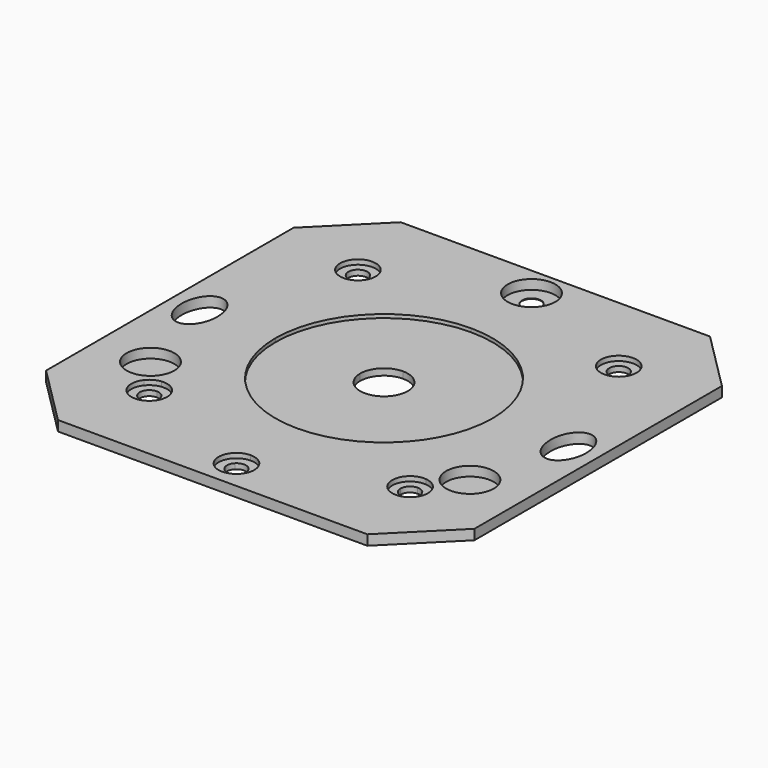
from build123d import *

# Parameters (mm, degrees)
F0_R      = 18.25
F1_DEPTH  = 1.7
F3_DEPTH  = 0.6
F4_R      = 1.6
F4_R_2    = 3
F5_DEPTH  = 0.8
F7_DEPTH  = 25
F8_R      = 2.5
F9_DEPTH  = 1.6
F10_R     = 4
F10_R_2   = 3
F11_DEPTH = 1.6
F13_DEPTH = 0.8
F15_DEPTH = 25


with BuildPart() as f1:
    # F0 (on Top) → F1 (new body)
    with BuildSketch(Plane.XY):
        Polygon((12.8613220751, 42.5075584586), (-39.1386779249, 42.5075584586), (-49.1386779249, 32.5075584586), (-49.1386779249, -19.4924415414), (-39.1386779249, -29.4924415414), (12.8613220751, -29.4924415414), (22.8613220751, -19.4924415414), (22.8613220751, 32.5075584586), align=None)
        with BuildLine():
            ThreePointArc((-35.0589881417, 26.8278686754), (-36.1903589916, 29.5592395253), (-33.4589881417, 28.4278686754))
            Line((-33.4589881417, 28.4278686754), (-22.2183677081, 28.4278686754))
            Line((-22.2183677081, 28.4278686754), (-14.2700487748, 36.3761876087))
            ThreePointArc((-14.2700487748, 36.3761876087), (-13.7509714167, 38.9857657106), (-11.5386779249, 37.5075584586))
            ThreePointArc((-11.5386779249, 37.5075584586), (-11.6604706729, 36.8952649668), (-12.007307075, 36.3761876087))
            Line((-12.007307075, 36.3761876087), (-4.0589881417, 28.4278686754))
            Line((-4.0589881417, 28.4278686754), (7.1816322919, 28.4278686754))
            ThreePointArc((7.1816322919, 28.4278686754), (8.7816322919, 30.0278686754), (10.3816322919, 28.4278686754))
            ThreePointArc((10.3816322919, 28.4278686754), (9.9130031418, 27.2964978255), (8.7816322919, 26.8278686754))
            Line((8.7816322919, 26.8278686754), (8.7816322919, 15.5872482418))
            Line((8.7816322919, 15.5872482418), (16.7299512252, 7.6389293085))
            ThreePointArc((16.7299512252, 7.6389293085), (18.4736155669, 7.9857657106), (19.4613220751, 6.5075584586))
            ThreePointArc((19.4613220751, 6.5075584586), (18.4736155669, 5.0293512066), (16.7299512252, 5.3761876087))
            Line((16.7299512252, 5.3761876087), (8.7816322919, -2.5721313246))
            Line((8.7816322919, -2.5721313246), (8.7816322919, -13.8127517582))
            ThreePointArc((8.7816322919, -13.8127517582), (9.9130031418, -14.2813809083), (10.3816322919, -15.4127517582))
            ThreePointArc((10.3816322919, -15.4127517582), (8.7816322919, -17.0127517582), (7.1816322919, -15.4127517582))
            Line((7.1816322919, -15.4127517582), (-4.0589881417, -15.4127517582))
            Line((-4.0589881417, -15.4127517582), (-12.007307075, -23.3610706915))
            ThreePointArc((-12.007307075, -23.3610706915), (-11.6604706729, -23.8801480496), (-11.5386779249, -24.4924415414))
            ThreePointArc((-11.5386779249, -24.4924415414), (-13.7509714167, -25.9706487934), (-14.2700487748, -23.3610706915))
            Line((-14.2700487748, -23.3610706915), (-22.2183677081, -15.4127517582))
            Line((-22.2183677081, -15.4127517582), (-33.4589881417, -15.4127517582))
            ThreePointArc((-33.4589881417, -15.4127517582), (-36.1903589916, -16.5441226081), (-35.0589881417, -13.8127517582))
            Line((-35.0589881417, -13.8127517582), (-35.0589881417, -2.5721313246))
            Line((-35.0589881417, -2.5721313246), (-43.007307075, 5.3761876087))
            ThreePointArc((-43.007307075, 5.3761876087), (-45.7386779249, 6.5075584586), (-43.007307075, 7.6389293085))
            Line((-43.007307075, 7.6389293085), (-35.0589881417, 15.5872482418))
            Line((-35.0589881417, 15.5872482418), (-35.0589881417, 26.8278686754))
        make_face(mode=Mode.SUBTRACT)
        with BuildLine():
            Line((-22.2183677081, 28.4278686754), (-33.4589881417, 28.4278686754))
            ThreePointArc((-33.4589881417, 28.4278686754), (-33.9276172918, 27.2964978255), (-35.0589881417, 26.8278686754))
            Line((-35.0589881417, 26.8278686754), (-35.0589881417, 15.5872482418))
            Line((-35.0589881417, 15.5872482418), (-22.2183677081, 28.4278686754))
        make_face()
        with BuildLine():
            Line((-14.2700487748, 36.3761876087), (-22.2183677081, 28.4278686754))
            Line((-22.2183677081, 28.4278686754), (-4.0589881417, 28.4278686754))
            Line((-4.0589881417, 28.4278686754), (-12.007307075, 36.3761876087))
            ThreePointArc((-12.007307075, 36.3761876087), (-13.1386779249, 35.9075584586), (-14.2700487748, 36.3761876087))
        make_face()
        with BuildLine():
            Line((7.1816322919, 28.4278686754), (-4.0589881417, 28.4278686754))
            Line((-4.0589881417, 28.4278686754), (8.7816322919, 15.5872482418))
            Line((8.7816322919, 15.5872482418), (8.7816322919, 26.8278686754))
            ThreePointArc((8.7816322919, 26.8278686754), (7.650261442, 27.2964978255), (7.1816322919, 28.4278686754))
        make_face()
        with BuildLine():
            Line((16.7299512252, 7.6389293085), (8.7816322919, 15.5872482418))
            Line((8.7816322919, 15.5872482418), (8.7816322919, -2.5721313246))
            Line((8.7816322919, -2.5721313246), (16.7299512252, 5.3761876087))
            ThreePointArc((16.7299512252, 5.3761876087), (16.2613220751, 6.5075584586), (16.7299512252, 7.6389293085))
        make_face()
        with BuildLine():
            Line((8.7816322919, -13.8127517582), (8.7816322919, -2.5721313246))
            Line((8.7816322919, -2.5721313246), (-4.0589881417, -15.4127517582))
            Line((-4.0589881417, -15.4127517582), (7.1816322919, -15.4127517582))
            ThreePointArc((7.1816322919, -15.4127517582), (7.650261442, -14.2813809083), (8.7816322919, -13.8127517582))
        make_face()
        with BuildLine():
            Line((-4.0589881417, -15.4127517582), (-22.2183677081, -15.4127517582))
            Line((-22.2183677081, -15.4127517582), (-14.2700487748, -23.3610706915))
            ThreePointArc((-14.2700487748, -23.3610706915), (-13.1386779249, -22.8924415414), (-12.007307075, -23.3610706915))
            Line((-12.007307075, -23.3610706915), (-4.0589881417, -15.4127517582))
        make_face()
        with BuildLine():
            Line((-22.2183677081, -15.4127517582), (-35.0589881417, -2.5721313246))
            Line((-35.0589881417, -2.5721313246), (-35.0589881417, -13.8127517582))
            ThreePointArc((-35.0589881417, -13.8127517582), (-33.9276172918, -14.2813809083), (-33.4589881417, -15.4127517582))
            Line((-33.4589881417, -15.4127517582), (-22.2183677081, -15.4127517582))
        make_face()
        with BuildLine():
            Line((-35.0589881417, -2.5721313246), (-35.0589881417, 15.5872482418))
            Line((-35.0589881417, 15.5872482418), (-43.007307075, 7.6389293085))
            ThreePointArc((-43.007307075, 7.6389293085), (-42.6604706729, 7.1198519504), (-42.5386779249, 6.5075584586))
            ThreePointArc((-42.5386779249, 6.5075584586), (-42.6604706729, 5.8952649668), (-43.007307075, 5.3761876087))
            Line((-43.007307075, 5.3761876087), (-35.0589881417, -2.5721313246))
        make_face()
        Polygon((-4.0589881417, 28.4278686754), (-22.2183677081, 28.4278686754), (-35.0589881417, 15.5872482418), (-35.0589881417, -2.5721313246), (-22.2183677081, -15.4127517582), (-4.0589881417, -15.4127517582), (8.7816322919, -2.5721313246), (8.7816322919, 15.5872482418), align=None)
        with Locations((-13.1386779249, 6.5075584586)):
            Circle(F0_R, mode=Mode.SUBTRACT)
        with Locations((-13.1386779249, 6.5075584586)):
            Circle(F0_R)
    extrude(amount=F1_DEPTH)

    # F2 (on face) → F3 (cut)
    with BuildSketch(Plane.XY.offset(1.7)):
        with BuildLine():
            Line((-31.3886779249, 6.5075584586), (-13.1386779249, 6.5075584586))
            Line((-13.1386779249, 6.5075584586), (-13.1386779249, 24.7575584586))
            ThreePointArc((-13.1386779249, 24.7575584586), (-26.0433766815, 19.4122572153), (-31.3886779249, 6.5075584586))
        make_face()
        with BuildLine():
            ThreePointArc((-13.1386779249, -11.7424415414), (-0.2339791682, -6.397140298), (5.1113220751, 6.5075584586))
            Line((5.1113220751, 6.5075584586), (-13.1386779249, 6.5075584586))
            Line((-13.1386779249, 6.5075584586), (-13.1386779249, -11.7424415414))
        make_face()
        with BuildLine():
            Line((-13.1386779249, 6.5075584586), (5.1113220751, 6.5075584586))
            ThreePointArc((5.1113220751, 6.5075584586), (-0.2339791682, 19.4122572153), (-13.1386779249, 24.7575584586))
            Line((-13.1386779249, 24.7575584586), (-13.1386779249, 6.5075584586))
        make_face()
        with BuildLine():
            Line((-13.1386779249, -11.7424415414), (-13.1386779249, 6.5075584586))
            Line((-13.1386779249, 6.5075584586), (-31.3886779249, 6.5075584586))
            ThreePointArc((-31.3886779249, 6.5075584586), (-26.0433766815, -6.397140298), (-13.1386779249, -11.7424415414))
        make_face()
    extrude(amount=-F3_DEPTH, mode=Mode.SUBTRACT)

    # F4 (on face) → F5 (cut)
    with BuildSketch(Plane.XY.offset(1.7)):
        with BuildLine():
            ThreePointArc((-45.7386779249, 6.5075584586), (-44.1386779249, 8.1075584586), (-42.5386779249, 6.5075584586))
            Line((-42.5386779249, 6.5075584586), (-41.1386779249, 6.5075584586))
            ThreePointArc((-41.1386779249, 6.5075584586), (-44.1386779249, 9.5075584586), (-47.1386779249, 6.5075584586))
            Line((-47.1386779249, 6.5075584586), (-45.7386779249, 6.5075584586))
        make_face()
        with BuildLine():
            ThreePointArc((-45.7386779249, 6.5075584586), (-44.1386779249, 4.9075584586), (-42.5386779249, 6.5075584586))
            Line((-42.5386779249, 6.5075584586), (-45.7386779249, 6.5075584586))
        make_face()
        with BuildLine():
            Line((-45.7386779249, 6.5075584586), (-42.5386779249, 6.5075584586))
            ThreePointArc((-42.5386779249, 6.5075584586), (-44.1386779249, 8.1075584586), (-45.7386779249, 6.5075584586))
        make_face()
        with BuildLine():
            Line((-41.1386779249, 6.5075584586), (-42.5386779249, 6.5075584586))
            ThreePointArc((-42.5386779249, 6.5075584586), (-44.1386779249, 4.9075584586), (-45.7386779249, 6.5075584586))
            Line((-45.7386779249, 6.5075584586), (-47.1386779249, 6.5075584586))
            ThreePointArc((-47.1386779249, 6.5075584586), (-44.1386779249, 3.5075584586), (-41.1386779249, 6.5075584586))
        make_face()
        with BuildLine():
            ThreePointArc((-35.4323567059, -9.5934317721), (-36.3209238445, -8.8312520534), (-37.4590547769, -8.5571581567))
            Line((-37.4590547769, -8.5571581567), (-37.4590547769, -11.0571581567))
            Line((-37.4590547769, -11.0571581567), (-35.4323567059, -9.5934317721))
        make_face()
        with BuildLine():
            Line((-37.4590547769, -11.0571581567), (-37.4590547769, -8.5571581567))
            ThreePointArc((-37.4590547769, -8.5571581567), (-39.6849608802, -9.9190272243), (-39.4857528479, -12.5208845413))
            Line((-39.4857528479, -12.5208845413), (-37.4590547769, -11.0571581567))
        make_face()
        with BuildLine():
            Line((-34.9590547769, -11.0571581567), (-37.4590547769, -11.0571581567))
            Line((-37.4590547769, -11.0571581567), (-39.4857528479, -12.5208845413))
            ThreePointArc((-39.4857528479, -12.5208845413), (-38.5779651724, -13.2927877161), (-37.4159766348, -13.5567869839))
            ThreePointArc((-37.4159766348, -13.5567869839), (-36.5068235367, -12.7852486338), (-35.3689396686, -12.4288063748))
            ThreePointArc((-35.3689396686, -12.4288063748), (-35.0637168288, -11.7729487089), (-34.9590547769, -11.0571581567))
        make_face()
        with BuildLine():
            Line((-35.4323567059, -9.5934317721), (-37.4590547769, -11.0571581567))
            Line((-37.4590547769, -11.0571581567), (-34.9590547769, -11.0571581567))
            ThreePointArc((-34.9590547769, -11.0571581567), (-35.0803213768, -10.2879849569), (-35.4323567059, -9.5934317721))
        make_face()
        with BuildLine():
            ThreePointArc((-35.3689396686, -12.4288063748), (-36.5068235367, -12.7852486338), (-37.4159766348, -13.5567869839))
            ThreePointArc((-37.4159766348, -13.5567869839), (-36.252525281, -13.2467440937), (-35.3689396686, -12.4288063748))
        make_face()
        with BuildLine():
            ThreePointArc((-35.3689396686, -12.4288063748), (-36.252525281, -13.2467440937), (-37.4159766348, -13.5567869839))
            ThreePointArc((-37.4159766348, -13.5567869839), (-36.0410865381, -18.2474444646), (-32.0589881417, -15.4127517582))
            ThreePointArc((-32.0589881417, -15.4127517582), (-33.0502391007, -13.1845400783), (-35.3689396686, -12.4288063748))
        make_face()
        with Locations((-35.0589881417, -15.4127517582)):
            Circle(F4_R, mode=Mode.SUBTRACT)
        with BuildLine():
            ThreePointArc((-13.1386779249, 40.5075584586), (-16.1386779249, 37.5075584586), (-13.1386779249, 34.5075584586))
            Line((-13.1386779249, 34.5075584586), (-13.1386779249, 35.9075584586))
            ThreePointArc((-13.1386779249, 35.9075584586), (-14.7386779249, 37.5075584586), (-13.1386779249, 39.1075584586))
            Line((-13.1386779249, 39.1075584586), (-13.1386779249, 40.5075584586))
        make_face()
        with BuildLine():
            Line((-13.1386779249, 35.9075584586), (-13.1386779249, 34.5075584586))
            ThreePointArc((-13.1386779249, 34.5075584586), (-11.0173575813, 35.3862381151), (-10.1386779249, 37.5075584586))
            ThreePointArc((-10.1386779249, 37.5075584586), (-11.0173575813, 39.6288788022), (-13.1386779249, 40.5075584586))
            Line((-13.1386779249, 40.5075584586), (-13.1386779249, 39.1075584586))
            ThreePointArc((-13.1386779249, 39.1075584586), (-12.007307075, 38.6389293085), (-11.5386779249, 37.5075584586))
            ThreePointArc((-11.5386779249, 37.5075584586), (-12.007307075, 36.3761876087), (-13.1386779249, 35.9075584586))
        make_face()
        with BuildLine():
            ThreePointArc((-10.1386779249, -24.4924415414), (-11.0173575813, -22.3711211978), (-13.1386779249, -21.4924415414))
            Line((-13.1386779249, -21.4924415414), (-13.1386779249, -22.8924415414))
            ThreePointArc((-13.1386779249, -22.8924415414), (-12.007307075, -23.3610706915), (-11.5386779249, -24.4924415414))
            ThreePointArc((-11.5386779249, -24.4924415414), (-12.007307075, -25.6238123913), (-13.1386779249, -26.0924415414))
            Line((-13.1386779249, -26.0924415414), (-13.1386779249, -27.4924415414))
            ThreePointArc((-13.1386779249, -27.4924415414), (-11.0173575813, -26.6137618849), (-10.1386779249, -24.4924415414))
        make_face()
        with BuildLine():
            Line((-13.1386779249, -22.8924415414), (-13.1386779249, -21.4924415414))
            ThreePointArc((-13.1386779249, -21.4924415414), (-16.1386779249, -24.4924415414), (-13.1386779249, -27.4924415414))
            Line((-13.1386779249, -27.4924415414), (-13.1386779249, -26.0924415414))
            ThreePointArc((-13.1386779249, -26.0924415414), (-14.7386779249, -24.4924415414), (-13.1386779249, -22.8924415414))
        make_face()
        with BuildLine():
            ThreePointArc((11.1816989271, -8.5571581567), (10.0435679947, -8.8312520534), (9.1550008561, -9.5934317721))
            Line((9.1550008561, -9.5934317721), (11.1816989271, -11.0571581567))
            Line((11.1816989271, -11.0571581567), (11.1816989271, -8.5571581567))
        make_face()
        with BuildLine():
            Line((11.1816989271, -11.0571581567), (9.1550008561, -9.5934317721))
            ThreePointArc((9.1550008561, -9.5934317721), (8.802965527, -10.2879849569), (8.6816989271, -11.0571581567))
            Line((8.6816989271, -11.0571581567), (11.1816989271, -11.0571581567))
        make_face()
        with BuildLine():
            ThreePointArc((20.8613220751, 6.5075584586), (17.8613220751, 9.5075584586), (14.8613220751, 6.5075584586))
            Line((14.8613220751, 6.5075584586), (16.2613220751, 6.5075584586))
            ThreePointArc((16.2613220751, 6.5075584586), (17.8613220751, 8.1075584586), (19.4613220751, 6.5075584586))
            Line((19.4613220751, 6.5075584586), (20.8613220751, 6.5075584586))
        make_face()
        with BuildLine():
            Line((16.2613220751, 6.5075584586), (14.8613220751, 6.5075584586))
            ThreePointArc((14.8613220751, 6.5075584586), (17.8613220751, 3.5075584586), (20.8613220751, 6.5075584586))
            Line((20.8613220751, 6.5075584586), (19.4613220751, 6.5075584586))
            ThreePointArc((19.4613220751, 6.5075584586), (17.8613220751, 4.9075584586), (16.2613220751, 6.5075584586))
        make_face()
        with BuildLine():
            ThreePointArc((13.6816989271, -11.0571581567), (12.9494658801, -9.2893912037), (11.1816989271, -8.5571581567))
            Line((11.1816989271, -8.5571581567), (11.1816989271, -11.0571581567))
            Line((11.1816989271, -11.0571581567), (13.2083969981, -12.5208845413))
            ThreePointArc((13.2083969981, -12.5208845413), (13.5604323272, -11.8263313565), (13.6816989271, -11.0571581567))
        make_face()
        with BuildLine():
            ThreePointArc((11.138620785, -13.5567869839), (10.229467687, -12.7852486338), (9.0915838189, -12.4288063748))
            ThreePointArc((9.0915838189, -12.4288063748), (9.9751694312, -13.2467440937), (11.138620785, -13.5567869839))
        make_face()
        with BuildLine():
            ThreePointArc((11.138620785, -13.5567869839), (9.9751694312, -13.2467440937), (9.0915838189, -12.4288063748))
            ThreePointArc((9.0915838189, -12.4288063748), (6.553420612, -17.4215007991), (11.7816322919, -15.4127517582))
            ThreePointArc((11.7816322919, -15.4127517582), (11.6163249983, -14.4306533617), (11.138620785, -13.5567869839))
        make_face()
        with Locations((8.7816322919, -15.4127517582)):
            Circle(F4_R, mode=Mode.SUBTRACT)
        with BuildLine():
            ThreePointArc((19.4613220751, 6.5075584586), (17.8613220751, 8.1075584586), (16.2613220751, 6.5075584586))
            Line((16.2613220751, 6.5075584586), (19.4613220751, 6.5075584586))
        make_face()
        with BuildLine():
            Line((19.4613220751, 6.5075584586), (16.2613220751, 6.5075584586))
            ThreePointArc((16.2613220751, 6.5075584586), (17.8613220751, 4.9075584586), (19.4613220751, 6.5075584586))
        make_face()
        with Locations((-35.0589881417, 28.4278686754)):
            Circle(F4_R_2)
        with Locations((-35.0589881417, 28.4278686754)):
            Circle(F4_R, mode=Mode.SUBTRACT)
        with Locations((8.7816322919, 28.4278686754)):
            Circle(F4_R_2)
        with Locations((8.7816322919, 28.4278686754)):
            Circle(F4_R, mode=Mode.SUBTRACT)
        with Locations((-35.0589881417, -15.4127517582)):
            Circle(F4_R)
        with Locations((8.7816322919, -15.4127517582)):
            Circle(F4_R)
        with Locations((-35.0589881417, 28.4278686754)):
            Circle(F4_R)
        with Locations((8.7816322919, 28.4278686754)):
            Circle(F4_R)
    extrude(amount=-F5_DEPTH, mode=Mode.SUBTRACT)

    # F6 (on face) → F7 (cut)
    with BuildSketch(Plane.XY.offset(1.7)):
        with BuildLine():
            ThreePointArc((-9.1386779249, 6.5075584586), (-10.3102508001, 9.3359855834), (-13.1386779249, 10.5075584586))
            Line((-13.1386779249, 10.5075584586), (-13.1386779249, 6.5075584586))
            Line((-13.1386779249, 6.5075584586), (-9.1386779249, 6.5075584586))
        make_face()
        with BuildLine():
            Line((-13.1386779249, 6.5075584586), (-13.1386779249, 10.5075584586))
            ThreePointArc((-13.1386779249, 10.5075584586), (-15.9671050496, 9.3359855834), (-17.1386779249, 6.5075584586))
            Line((-17.1386779249, 6.5075584586), (-13.1386779249, 6.5075584586))
        make_face()
        with BuildLine():
            Line((-9.1386779249, 6.5075584586), (-13.1386779249, 6.5075584586))
            Line((-13.1386779249, 6.5075584586), (-13.1386779249, 2.5075584586))
            ThreePointArc((-13.1386779249, 2.5075584586), (-10.3102508001, 3.6791313339), (-9.1386779249, 6.5075584586))
        make_face()
        with BuildLine():
            Line((-13.1386779249, 2.5075584586), (-13.1386779249, 6.5075584586))
            Line((-13.1386779249, 6.5075584586), (-17.1386779249, 6.5075584586))
            ThreePointArc((-17.1386779249, 6.5075584586), (-15.9671050496, 3.6791313339), (-13.1386779249, 2.5075584586))
        make_face()
    extrude(amount=-F7_DEPTH, mode=Mode.SUBTRACT)

    # F8 (on face) → F9 (join)
    with BuildSketch(Plane.XY.offset(1.7)):
        with Locations((-37.4590547769, -11.0571581567)):
            Circle(F8_R)
        with Locations((11.1816989271, -11.0571581567)):
            Circle(F8_R)
    extrude(amount=-F9_DEPTH)

    # F10 (on face) → F11 (cut)
    with BuildSketch(Plane.XY.offset(1.7)):
        with Locations((-13.1386779249, 37.5075584586)):
            Circle(F10_R)
        with Locations((-13.1386779249, 37.5075584586)):
            Circle(F10_R_2, mode=Mode.SUBTRACT)
        with Locations((13.7081095924, -8.9924415414)):
            Circle(F10_R)
        with Locations((-39.9854654422, -8.9924415414)):
            Circle(F10_R)
        with Locations((-44.1386779249, 6.5075584586)):
            Circle(F10_R_2)
        with Locations((-13.1386779249, 37.5075584586)):
            Circle(F10_R_2)
    extrude(amount=-F11_DEPTH, mode=Mode.SUBTRACT)

    # F12 (on face) → F13 (cut)
    with BuildSketch(Plane.XY.offset(1.7)):
        with BuildLine():
            ThreePointArc((9.0915838189, -12.4288063748), (9.9751694312, -13.2467440937), (11.138620785, -13.5567869839))
            ThreePointArc((11.138620785, -13.5567869839), (10.229467687, -12.7852486338), (9.0915838189, -12.4288063748))
        make_face()
        with BuildLine():
            ThreePointArc((9.0915838189, -12.4288063748), (6.553420612, -17.4215007991), (11.7816322919, -15.4127517582))
            ThreePointArc((11.7816322919, -15.4127517582), (11.6163249983, -14.4306533617), (11.138620785, -13.5567869839))
            ThreePointArc((11.138620785, -13.5567869839), (9.9751694312, -13.2467440937), (9.0915838189, -12.4288063748))
        make_face()
        with BuildLine():
            ThreePointArc((-37.4159766348, -13.5567869839), (-36.0410865381, -18.2474444646), (-32.0589881417, -15.4127517582))
            ThreePointArc((-32.0589881417, -15.4127517582), (-33.0502391007, -13.1845400783), (-35.3689396686, -12.4288063748))
            ThreePointArc((-35.3689396686, -12.4288063748), (-36.252525281, -13.2467440937), (-37.4159766348, -13.5567869839))
        make_face()
        with BuildLine():
            ThreePointArc((-37.4159766348, -13.5567869839), (-36.252525281, -13.2467440937), (-35.3689396686, -12.4288063748))
            ThreePointArc((-35.3689396686, -12.4288063748), (-36.5068235367, -12.7852486338), (-37.4159766348, -13.5567869839))
        make_face()
    extrude(amount=-F13_DEPTH, mode=Mode.SUBTRACT)

    # F14 (on face) → F15 (cut)
    with BuildSketch(Plane.XY.offset(1.7)):
        with BuildLine():
            add(Edge.make_bspline(
                [(-47.1386779249, 6.5075585663), (-47.1386779967, 2.0075585125), (-44.1386779608, 2.0075584586), (-41.1386779249, 2.0075584048), (-41.1386779249, 6.5075584586)],
                knots=[1.5707963029, 1.5707963029, 1.5707963029, 3.1415926416, 3.1415926416, 4.7123889804, 4.7123889804, 4.7123889804], degree=2, weights=[1, 0.707106777, 1, 0.707106777, 1]))
            ThreePointArc((-41.1386779249, 6.5075584586), (-44.1386779787, 3.5075584586), (-47.1386779249, 6.5075585663))
        make_face()
        with BuildLine():
            add(Edge.make_bspline(
                [(14.8613220751, 6.5075584586), (14.8613220751, 2.0075584586), (17.8613220751, 2.0075584586), (20.8613220751, 2.0075584586), (20.8613220751, 6.5075584586)],
                knots=[1.5707963268, 1.5707963268, 1.5707963268, 3.1415926536, 3.1415926536, 4.7123889804, 4.7123889804, 4.7123889804], degree=2, weights=[1, 0.7071067812, 1, 0.7071067812, 1]))
            ThreePointArc((20.8613220751, 6.5075584586), (17.8613220751, 3.5075584586), (14.8613220751, 6.5075584586))
        make_face()
        with BuildLine():
            ThreePointArc((14.8613220751, 6.5075584586), (17.8613220751, 9.5075584586), (20.8613220751, 6.5075584586))
            add(Edge.make_bspline(
                [(20.8613220751, 6.5075584586), (20.8613220751, 11.0075584586), (17.8613220751, 11.0075584586)],
                knots=[4.7123889804, 4.7123889804, 4.7123889804, 6.2831853072, 6.2831853072, 6.2831853072], degree=2, weights=[1, 0.7071067812, 1]))
            add(Edge.make_bspline(
                [(17.8613220751, 11.0075584586), (14.8613220751, 11.0075584586), (14.8613220751, 6.5075584586)],
                knots=[0, 0, 0, 1.5707963268, 1.5707963268, 1.5707963268], degree=2, weights=[1, 0.7071067812, 1]))
        make_face()
        with BuildLine():
            ThreePointArc((-47.1386779249, 6.5075585663), (-44.1386779787, 3.5075584586), (-41.1386779249, 6.5075584586))
            ThreePointArc((-41.1386779249, 6.5075584586), (-44.138677871, 9.5075584586), (-47.1386779249, 6.5075585663))
        make_face()
        with BuildLine():
            ThreePointArc((14.8613220751, 6.5075584586), (17.8613220751, 3.5075584586), (20.8613220751, 6.5075584586))
            ThreePointArc((20.8613220751, 6.5075584586), (17.8613220751, 9.5075584586), (14.8613220751, 6.5075584586))
        make_face()
        with BuildLine():
            ThreePointArc((-47.1386779249, 6.5075585663), (-44.138677871, 9.5075584586), (-41.1386779249, 6.5075584586))
            add(Edge.make_bspline(
                [(-41.1386779249, 6.5075584586), (-41.1386779249, 11.0075584586), (-44.1386779249, 11.0075584586)],
                knots=[4.7123889804, 4.7123889804, 4.7123889804, 6.2831853072, 6.2831853072, 6.2831853072], degree=2, weights=[1, 0.7071067812, 1]))
            add(Edge.make_bspline(
                [(-44.1386779249, 11.0075584586), (-47.1386778531, 11.0075584586), (-47.1386779249, 6.5075585663)],
                knots=[0, 0, 0, 1.5707963029, 1.5707963029, 1.5707963029], degree=2, weights=[1, 0.7071067896, 1]))
        make_face()
    extrude(amount=-F15_DEPTH, mode=Mode.SUBTRACT)


solid = f1.part
